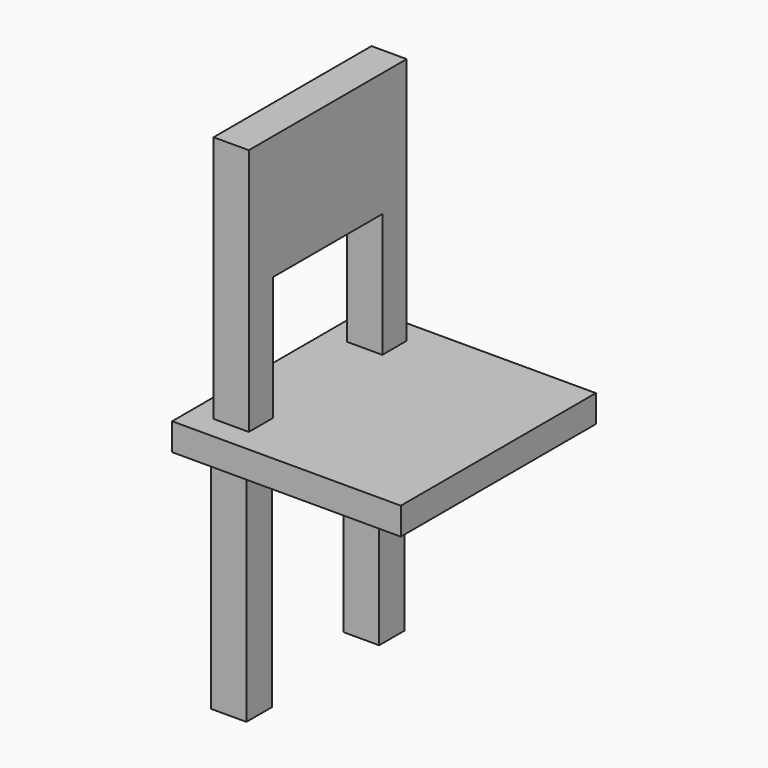
from build123d import *

# Parameters (mm, degrees)
F0_W      = 106.4638644457
F0_H      = 103.2169535756
F1_DEPTH  = 12.7
F2_W      = 16.3826718926
F2_H      = 14.1792520881
F3_DEPTH  = 115.4824048281
F4_W      = 16.3826718926
F4_H      = 57.741202414
F5_DEPTH  = 25.4
F7_DEPTH  = 12.7457336903
F8_W      = 16.5637210011
F8_H      = 14.8448646069
F9_DEPTH  = 106.4620614052
F10_R     = 29.9454441035
F11_DEPTH = 25.4


with BuildPart() as f1:
    # F0 (on Top) → F1 (new body)
    with BuildSketch(Plane.XY):
        with Locations((3.0183121562, -5.1516257226)):
            Rectangle(F0_W, F0_H)
    extrude(amount=F1_DEPTH)

    # F2 (on face) → F3 (join)
    with BuildSketch(Plane.XY.offset(12.7)):
        with Locations((-31.3676968217, -38.8624928892)):
            Rectangle(F2_W, F2_H)
    extrude(amount=F3_DEPTH)

    # F4 (on face) → F5 (join)
    with BuildSketch(Plane(origin=(0, -31.7728668451, 0), x_dir=(-1, 0, 0), z_dir=(0, 1, 0))):
        with Locations((31.3676968217, 99.3118036211)):
            Rectangle(F4_W, F4_H)
    extrude(amount=F5_DEPTH)

    # F6: F1 across plane


with BuildPart() as f1_1:
    add(f1.part)
    add(f1.part.mirror(Plane.XZ))

    # F7 (add, through all): a face of the model
    f7_faces = [f1_1.faces().sort_by_distance(p)[0] for p in [
        (-31.3676968217, -6.3728668451, 99.3118036211),
    ]]
    extrude(f7_faces, amount=F7_DEPTH)

    # F8 (on face) → F9 (join)
    with BuildSketch(Plane(origin=(0, 0, 0), x_dir=(1, 0, 0), z_dir=(0, 0, -1))):
        with Locations((-32.4887447059, 38.6229231954)):
            Rectangle(F8_W, F8_H)
    extrude(amount=F9_DEPTH)

    # F13: F1 across plane


with BuildPart() as f11:
    # F10 (on Top) → F11 (new body)
    with BuildSketch(Plane.XY):
        with Locations((108.9618206024, 20.2722847462)):
            Circle(F10_R)
    extrude(amount=F11_DEPTH)


with BuildPart() as f1_2:
    add(f1_1.part)
    add(f1_1.part.mirror(Plane.XZ))


solid = f1_2.part
